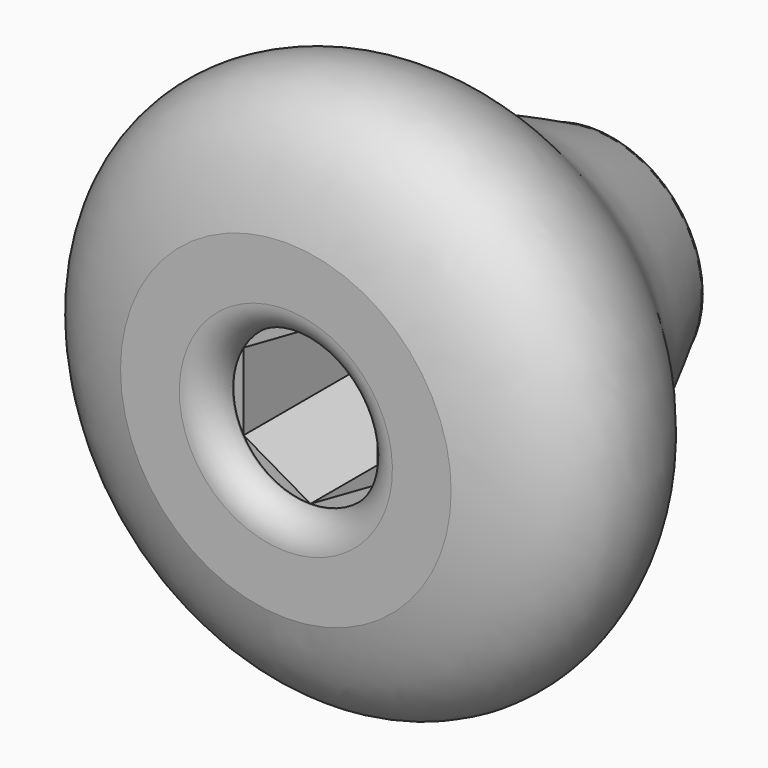
from build123d import *

# Parameters (mm, degrees)
F0_R     = 9.525
F1_DEPTH = 15.24
F3_DEPTH = 8.89
F4_R     = 3.683
F5_DEPTH = 6.351
F8_R     = 2.54
F9_DEPTH = 15.24


# Not quite as in the source:
# - a feature names something its author has since deleted; it is built from what else it names


with BuildPart() as f1:
    # F0 (on Front) → F1 (new body)
    with BuildSketch(Plane.XZ):
        Circle(F0_R)
    extrude(amount=F1_DEPTH)

    # F2 (on face) → F3 (cut)
    with BuildSketch(Plane.XZ.offset(15.24)):
        Polygon((5.7785, -3.3362185305), (5.7785, 3.3362185305), (0, 6.672437061), (-5.7785, 3.3362185305), (-5.7785, -3.3362185305), (0, -6.672437061), align=None)
    extrude(amount=-F3_DEPTH, mode=Mode.SUBTRACT)

    # F4 (on face) → F5 (cut, through all)
    with BuildSketch(Plane.XZ.offset(6.35)):
        Circle(F4_R)
    extrude(amount=-F5_DEPTH, mode=Mode.SUBTRACT)

    # F6 (on Right) → F7 (revolve)
    with BuildSketch(Plane.YZ):
        with BuildLine():
            Line((-33.139064908, -6.672437061), (-33.139064908, -14.292437061))
            add(Edge.make_bspline(
                [(0, -9.4667123631), (-6.0169453004, -12.6291806394), (-11.4998287108, -14.4075187704), (-18.7425000775, -24.446910043), (-30.9530390066, -25.1909209173), (-33.139064908, -14.292437061)],
                knots=[0, 0, 0, 0, 0.3337672016, 0.635034675, 1, 1, 1, 1], degree=3))
            Line((0, -9.4667123631), (0, -6.672437061))
            Line((0, -6.672437061), (-33.139064908, -6.672437061))
        make_face()
    revolve(axis=Axis((0, -11.1619029194, 0), (0, -1, 0)))

    # F8
    f8_edges = [f1.edges().sort_by_distance(p)[0] for p in [
        (0, -33.139065, 6.672437),
    ]]
    fillet(f8_edges, radius=F8_R)

    # F9 (add): faces of the model
    f9_faces = [f1.faces().sort_by_distance(p)[0] for p in [
        (-3.069105432, -15.24, 5.315846542),
        (-6.138210864, -15.24, 0),
        (-3.069105432, -15.24, -5.315846542),
        (6.138210864, -15.24, 0),
        (3.069105432, -15.24, -5.315846542),
        (3.069105432, -15.24, 5.315846542),
    ]]
    extrude(f9_faces, amount=F9_DEPTH)


solid = f1.part
